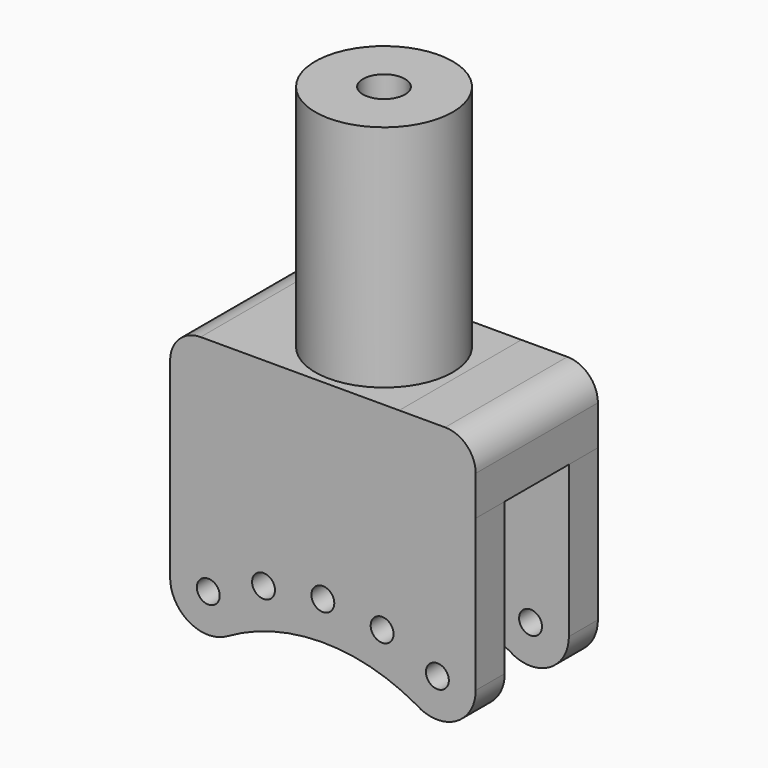
from build123d import *

# Parameters (mm, degrees)
F0_R     = 1.5
F1_DEPTH = 10
F2_DEPTH = 5.25
F3_R     = 9
F3_R_2   = 7
F3_R_3   = 2.75
F4_DEPTH = 30
F5_DEPTH = 8.8
F6_DEPTH = 5.0771655029


# Not quite as in the source:
# - ends of sketch curves that miss each other by under 0.0002 mm in the source are joined


with BuildPart() as f1:
    # F0 (on Front) → F1 (new body, symmetric)
    with BuildSketch(Plane.XZ):
        with BuildLine():
            ThreePointArc((20.0087781194, -9.6635037267), (10.2175079385, -6.5385316067), (-0.005862, -5.4815880859))
            ThreePointArc((-0.005862, -5.4815880859), (-10.2228373041, -6.5359722724), (-20.0087868417, -9.6558283627))
            Line((-20.0087868417, -9.6558283627), (-20.008784, -29.496459))
            Line((-20.008784, -29.496459), (-20.008784, -29.500828))
            ThreePointArc((-20.008784, -29.500828), (-17.5087901054, -33.8309491846), (-12.5087967107, -33.8309485011))
            ThreePointArc((-12.5087967107, -33.8309485011), (-0.2003110708, -30.4823215942), (12.1580317725, -33.6419823498))
            ThreePointArc((12.1580317725, -33.6419823498), (12.4912575647, -33.830982099), (12.8215481384, -34.0250657685))
            ThreePointArc((12.8215481384, -34.0250657685), (17.6641901361, -33.7471454023), (20.008785, -29.500824))
            Line((20.008785, -29.500824), (20.0087781194, -9.6635037267))
        make_face()
        with Locations((-15.008794, -29.500828)):
            Circle(F0_R, mode=Mode.SUBTRACT)
        with Locations((-7.773364, -26.503811)):
            Circle(F0_R, mode=Mode.SUBTRACT)
        with BuildLine():
            ThreePointArc((-0.008573175, -23.9815880161), (1.0519448888, -24.4210055509), (1.491207, -25.481588))
            ThreePointArc((1.491207, -25.481588), (-1.0695308888, -26.5421704491), (-0.008573175, -23.9815880161))
        make_face(mode=Mode.SUBTRACT)
        with Locations((7.755782, -26.503815)):
            Circle(F0_R, mode=Mode.SUBTRACT)
        with Locations((14.991208, -29.500824)):
            Circle(F0_R, mode=Mode.SUBTRACT)
        with BuildLine():
            Line((-0.0051292502, -0.48159), (-0.0058619999, -5.4815880859))
            ThreePointArc((-0.0058619999, -5.4815880859), (10.2175079385, -6.5385316067), (20.0087781194, -9.6635037267))
            Line((20.0087781194, -9.6635037267), (20.008783, -4.481588))
            ThreePointArc((20.008783, -4.481588), (18.8372111247, -1.6531608753), (16.008784, -0.481588))
            Line((16.008784, -0.481588), (9.991212, -0.48159))
            Line((9.991212, -0.48159), (-0.0051292502, -0.48159))
        make_face()
        with BuildLine():
            ThreePointArc((-20.0087868417, -9.6558283627), (-10.2228373041, -6.5359722724), (-0.005862, -5.4815880859))
            Line((-0.005862, -5.4815880859), (-0.0051292502, -0.48159))
            Line((-0.0051292502, -0.48159), (-10.008792, -0.48159))
            Line((-10.008792, -0.48159), (-16.008784, -0.48159))
            ThreePointArc((-16.008784, -0.48159), (-18.8372111247, -1.6531608753), (-20.008784, -4.481588))
            Line((-20.008784, -4.481588), (-20.0087868417, -9.6558283627))
        make_face()
    extrude(amount=F1_DEPTH, both=True)

    # F0 (on Front) → F2 (cut, symmetric)
    with BuildSketch(Plane.XZ):
        with BuildLine():
            ThreePointArc((20.0087781194, -9.6635037267), (10.2175079385, -6.5385316067), (-0.005862, -5.4815880859))
            ThreePointArc((-0.005862, -5.4815880859), (-10.2228373041, -6.5359722724), (-20.0087868417, -9.6558283627))
            Line((-20.0087868417, -9.6558283627), (-20.008784, -29.496459))
            Line((-20.008784, -29.496459), (-20.008784, -29.500828))
            ThreePointArc((-20.008784, -29.500828), (-17.5087901054, -33.8309491846), (-12.5087967107, -33.8309485011))
            ThreePointArc((-12.5087967107, -33.8309485011), (-0.2003110708, -30.4823215942), (12.1580317725, -33.6419823498))
            ThreePointArc((12.1580317725, -33.6419823498), (12.4912575647, -33.830982099), (12.8215481384, -34.0250657685))
            ThreePointArc((12.8215481384, -34.0250657685), (17.6641901361, -33.7471454023), (20.008785, -29.500824))
            Line((20.008785, -29.500824), (20.0087781194, -9.6635037267))
        make_face()
        with Locations((-15.008794, -29.500828)):
            Circle(F0_R, mode=Mode.SUBTRACT)
        with Locations((-7.773364, -26.503811)):
            Circle(F0_R, mode=Mode.SUBTRACT)
        with BuildLine():
            ThreePointArc((-0.008573175, -23.9815880161), (1.0519448888, -24.4210055509), (1.491207, -25.481588))
            ThreePointArc((1.491207, -25.481588), (-1.0695308888, -26.5421704491), (-0.008573175, -23.9815880161))
        make_face(mode=Mode.SUBTRACT)
        with Locations((7.755782, -26.503815)):
            Circle(F0_R, mode=Mode.SUBTRACT)
        with Locations((14.991208, -29.500824)):
            Circle(F0_R, mode=Mode.SUBTRACT)
    extrude(amount=F2_DEPTH, both=True, mode=Mode.SUBTRACT)

    # F3 (on face) → F4 (join)
    with BuildSketch(Plane.XY.offset(-0.48159)):
        Circle(F3_R)
        Circle(F3_R_2, mode=Mode.SUBTRACT)
        Circle(F3_R_2)
        Polygon((3.8423572259, 2.4575647055), (4.0494920794, -2.0987966153), (0.2071348534, -4.5563613208), (-3.8423572259, -2.4575647055), (-4.0494920794, 2.0987966153), (-0.2071348534, 4.5563613208), align=None, mode=Mode.SUBTRACT)
        Polygon((0.2071348534, -4.5563613208), (4.0494920794, -2.0987966153), (3.8423572259, 2.4575647055), (-0.2071348534, 4.5563613208), (-4.0494920794, 2.0987966153), (-3.8423572259, -2.4575647055), align=None)
        Circle(F3_R_3, mode=Mode.SUBTRACT)
    extrude(amount=F4_DEPTH)

    # F3 (on face) → F5 (join)
    with BuildSketch(Plane.XY.offset(-0.48159)):
        Circle(F3_R_2)
        Polygon((3.8423572259, 2.4575647055), (4.0494920794, -2.0987966153), (0.2071348534, -4.5563613208), (-3.8423572259, -2.4575647055), (-4.0494920794, 2.0987966153), (-0.2071348534, 4.5563613208), align=None, mode=Mode.SUBTRACT)
    extrude(amount=-F5_DEPTH)

    # F3 (on face) → F6 (cut, through all)
    with BuildSketch(Plane.XY.offset(-0.48159)):
        Circle(F3_R_3)
    extrude(amount=-F6_DEPTH, mode=Mode.SUBTRACT)


solid = f1.part
